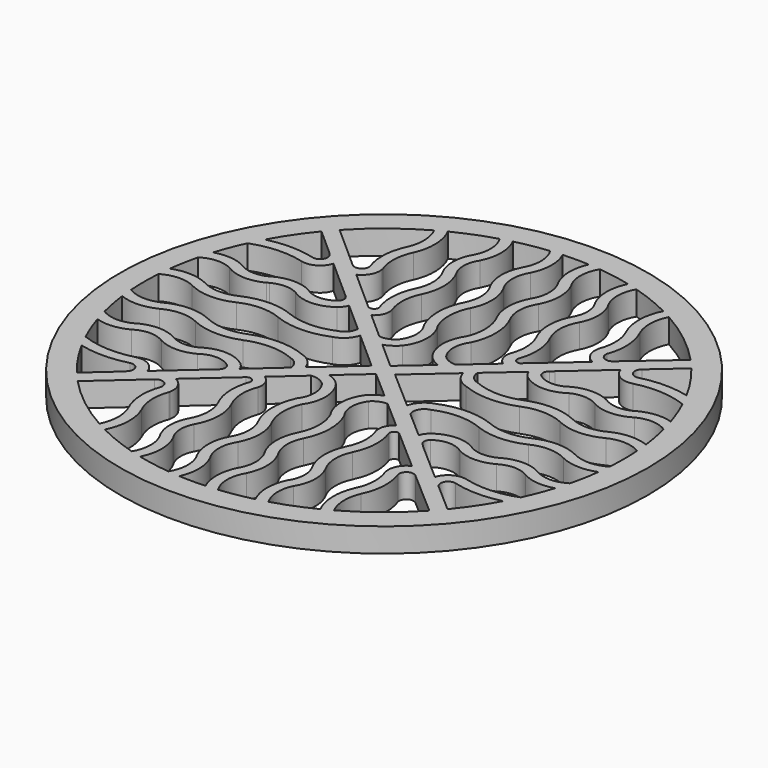
from build123d import *

# Parameters (mm, degrees)
F0_R     = 27.94
F1_DEPTH = 2.54


# Not quite as in the source:
# - ends of sketch curves that miss each other by under 0.0002 mm in the source are joined


with BuildPart() as f1:
    # F0 (on Top) → F1 (new body)
    with BuildSketch(Plane.XY):
        Circle(F0_R)
        with BuildLine():
            Line((-18.5704831808, -17.3290840621), (-13.8005321379, -13.098635549))
            ThreePointArc((-13.8005321379, -13.098635549), (-12.906008286, -13.0112132814), (-12.5460925989, -13.8347885801))
            ThreePointArc((-12.5460925989, -13.8347885801), (-12.8977992847, -16.1722814952), (-12.3113500616, -18.4621828096))
            ThreePointArc((-12.3113500616, -18.4621828096), (-11.9533208933, -20.3219772897), (-12.4161624395, -22.1584952169))
            ThreePointArc((-12.4161624395, -22.1584952169), (-15.6803652612, -19.9821456624), (-18.5704831808, -17.3290840621))
        make_face(mode=Mode.SUBTRACT)
        with BuildLine():
            Line((-16.5311535001, -13.4369904456), (-16.6220914229, -13.564037606))
            Line((-16.6220914229, -13.564037606), (-19.5763440963, -16.1841512543))
            ThreePointArc((-19.5763440963, -16.1841512543), (-21.0445692163, -14.2227320336), (-22.3169864748, -12.1289783034))
            ThreePointArc((-22.3169864748, -12.1289783034), (-19.7773206943, -12.4353403441), (-17.2424184103, -12.0917848367))
            ThreePointArc((-17.2424184103, -12.0917848367), (-16.3555594533, -12.4835065865), (-16.5311535001, -13.4369904456))
        make_face(mode=Mode.SUBTRACT)
        with BuildLine():
            Line((-12.4929334647, -11.9389320609), (-8.1518250801, -8.0888222075))
            ThreePointArc((-8.1518250801, -8.0888222075), (-7.5848144389, -8.0278903633), (-7.3414510498, -8.5436306251))
            ThreePointArc((-7.3414510498, -8.5436306251), (-7.6962049281, -10.8285786216), (-7.1160036617, -13.0669271539))
            ThreePointArc((-7.1160036617, -13.0669271539), (-6.7161500742, -14.9429747655), (-7.2321257599, -16.7904613349))
            ThreePointArc((-7.2321257599, -16.7904613349), (-7.7064237742, -18.845016734), (-7.0859523066, -20.8602516215))
            ThreePointArc((-7.0859523066, -20.8602516215), (-6.7211428867, -22.6227957974), (-7.2321257599, -24.3486417895))
            ThreePointArc((-7.2321257599, -24.3486417895), (-9.3559303924, -23.6141179486), (-11.4065002981, -22.6947516168))
            ThreePointArc((-11.4065002981, -22.6947516168), (-10.8107716851, -20.3540767822), (-11.2731624395, -17.9834553338))
            ThreePointArc((-11.2731624395, -17.9834553338), (-11.758060909, -16.0759793316), (-11.437578849, -14.1341033124))
            Line((-11.437578849, -14.1341033124), (-11.4188391308, -14.0269326452))
            ThreePointArc((-11.4188391308, -14.0269326452), (-11.596606163, -12.7981140346), (-12.4929334647, -11.9389320609))
        make_face(mode=Mode.SUBTRACT)
        with BuildLine():
            Line((-6.9854120479, -7.0543356408), (-4.1093686564, -4.5035854592))
            ThreePointArc((-4.1093686564, -4.5035854592), (-3.2193987681, -4.622483985), (-2.4732761203, -5.1219679745))
            ThreePointArc((-2.4732761203, -5.1219679745), (-1.9512402498, -6.7679594308), (-2.4983765115, -8.4057784791))
            ThreePointArc((-2.4983765115, -8.4057784791), (-3.0543737307, -11.0452272125), (-2.4107500728, -13.6646872925))
            ThreePointArc((-2.4107500728, -13.6646872925), (-2.0125173354, -15.4777115994), (-2.5659752822, -17.2495272647))
            ThreePointArc((-2.5659752822, -17.2495272647), (-3.0984296295, -19.3613287647), (-2.6085446443, -21.4834093261))
            ThreePointArc((-2.6085446443, -21.4834093261), (-2.088534568, -23.3762023641), (-2.6272335105, -25.2637614793))
            ThreePointArc((-2.6272335105, -25.2637614793), (-4.3733190571, -25.020673061), (-6.0983371667, -24.657053429))
            ThreePointArc((-6.0983371667, -24.657053429), (-6.0937218208, -24.6479307461), (-6.0891257599, -24.638798332))
            ThreePointArc((-6.0891257599, -24.638798332), (-5.5749024675, -22.4680644679), (-6.0891257599, -20.2973306037))
            ThreePointArc((-6.0891257599, -20.2973306037), (-6.5627915104, -18.8369130713), (-6.2289017722, -17.3383483398))
            ThreePointArc((-6.2289017722, -17.3383483398), (-5.5734089799, -14.9687958695), (-6.0891257599, -12.5649477228))
            ThreePointArc((-6.0891257599, -12.5649477228), (-6.5561181002, -10.7393618485), (-6.2466127495, -8.8805848129))
            ThreePointArc((-6.2466127495, -8.8805848129), (-6.3100290028, -7.8436762867), (-6.9854120479, -7.0543356408))
        make_face(mode=Mode.SUBTRACT)
        with BuildLine():
            Line((-10.7794748619, -8.3822467826), (-15.2007910101, -12.3034925472))
            ThreePointArc((-15.2007910101, -12.3034925472), (-16.1010101713, -11.1724173912), (-17.5346267563, -10.9867590113))
            ThreePointArc((-17.5346267563, -10.9867590113), (-20.3062535778, -11.2809984553), (-23.0334956908, -10.7059831993))
            ThreePointArc((-23.0334956908, -10.7059831993), (-23.6783363344, -9.19219171), (-24.2238119338, -7.639825613))
            ThreePointArc((-24.2238119338, -7.639825613), (-22.5093516319, -7.8291197338), (-20.856343234, -7.3364031546))
            ThreePointArc((-20.856343234, -7.3364031546), (-19.2961519486, -6.8658747452), (-17.7295057945, -7.3144432007))
            ThreePointArc((-17.7295057945, -7.3144432007), (-15.8135280217, -7.7981545882), (-13.8921396836, -7.3364031546))
            ThreePointArc((-13.8921396836, -7.3364031546), (-12.3358072727, -6.8157514758), (-10.7794748619, -7.3364031546))
            ThreePointArc((-10.7794748619, -7.3364031546), (-10.5312463908, -7.8303040534), (-10.7360509039, -8.3437342659))
            ThreePointArc((-10.7360509039, -8.3437342659), (-10.7573480268, -8.3634582863), (-10.7794748619, -8.3822467826))
        make_face(mode=Mode.SUBTRACT)
        with BuildLine():
            ThreePointArc((-24.6333464508, -6.1934031546), (-24.9649839092, -4.6807668616), (-25.2038268228, -3.1507322145))
            ThreePointArc((-25.2038268228, -3.1507322145), (-23.2746663282, -3.4703434645), (-21.3780211987, -2.994372018))
            ThreePointArc((-21.3780211987, -2.994372018), (-19.501415105, -2.5043500763), (-17.6065823104, -2.9183314944))
            ThreePointArc((-17.6065823104, -2.9183314944), (-15.0565101754, -3.5137315462), (-12.4770380559, -3.0624082698))
            ThreePointArc((-12.4770380559, -3.0624082698), (-9.9451402811, -2.5677176934), (-7.4211004148, -3.1010542307))
            ThreePointArc((-7.4211004148, -3.1010542307), (-6.6509483041, -3.5810685005), (-6.317788309, -4.4251966842))
            Line((-6.317788309, -4.4251966842), (-9.495253242, -7.2432762998))
            ThreePointArc((-9.495253242, -7.2432762998), (-9.7298232295, -6.7980281825), (-10.0775378412, -6.4342102148))
            Line((-10.0775378412, -6.4342102148), (-10.0916950959, -6.4234913333))
            ThreePointArc((-10.0916950959, -6.4234913333), (-12.2793958042, -5.673178142), (-14.4887914077, -6.3569729516))
            ThreePointArc((-14.4887914077, -6.3569729516), (-15.9583042621, -6.6504710139), (-17.3854335884, -6.1934031546))
            ThreePointArc((-17.3854335884, -6.1934031546), (-19.4293945717, -5.7257275396), (-21.4318401679, -6.3475865402))
            ThreePointArc((-21.4318401679, -6.3475865402), (-23.0532754063, -6.6999436052), (-24.6333464508, -6.1934031546))
        make_face(mode=Mode.SUBTRACT)
        with BuildLine():
            Line((-3.0008579849, -3.4897487406), (-0.1074668487, -0.9299076392))
            Line((-0.1074668487, -0.9299076392), (2.8724846558, -3.5323386056))
            ThreePointArc((2.8724846558, -3.5323386056), (2.1752585082, -3.8839965102), (1.5870080755, -4.397561512))
            ThreePointArc((1.5870080755, -4.397561512), (0.8087695638, -6.6735323176), (1.5017849321, -8.9768837863))
            ThreePointArc((1.5017849321, -8.9768837863), (1.9103804325, -11.0743224779), (1.3914487995, -13.1472212473))
            ThreePointArc((1.3914487995, -13.1472212473), (1.3803900845, -13.1691739034), (1.3692218584, -13.1910710497))
            ThreePointArc((1.3692218584, -13.1910710497), (0.8667364927, -15.4065827451), (1.4482800878, -17.602668049))
            Line((1.4482800878, -17.602668049), (1.4530981237, -17.6022709756))
            ThreePointArc((1.4530981237, -17.6022709756), (1.955462941, -19.4080288753), (1.4530232551, -21.2137659447))
            ThreePointArc((1.4530232551, -21.2137659447), (0.9458843119, -23.2802576622), (1.385342962, -25.3621928247))
            ThreePointArc((1.385342962, -25.3621928247), (-0.0001316396, -25.3999999997), (-1.3856058492, -25.3621784638))
            ThreePointArc((-1.3856058492, -25.3621784638), (-0.9461256192, -23.2802478565), (-1.4532431425, -21.2137508825))
            ThreePointArc((-1.4532431425, -21.2137508825), (-1.9554739954, -19.3715116674), (-1.4149317469, -17.5401473582))
            ThreePointArc((-1.4149317469, -17.5401473582), (-0.8661983565, -15.3465313443), (-1.3915850746, -13.1472068237))
            ThreePointArc((-1.3915850746, -13.1472068237), (-1.9104952213, -11.0743026756), (-1.5018779803, -8.9768682194))
            ThreePointArc((-1.5018779803, -8.9768682194), (-0.8088387371, -6.6735239341), (-1.5870536575, -4.3975450619))
            ThreePointArc((-1.5870536575, -4.3975450619), (-2.2317910283, -3.8468312927), (-3.0008579849, -3.4897487406))
        make_face(mode=Mode.SUBTRACT)
        with BuildLine():
            ThreePointArc((-7.0508121213, 2.0164165737), (-6.0285782094, 2.6143373536), (-5.4245050427, 3.6329477006))
            Line((-5.4245050427, 3.6329477006), (-1.328253163, 0))
            Line((-1.328253163, 0), (-5.4245050427, -3.6329477006))
            ThreePointArc((-5.4245050427, -3.6329477006), (-6.0285782094, -2.6143373536), (-7.0508121213, -2.0164165737))
            ThreePointArc((-7.0508121213, -2.0164165737), (-9.9151064709, -1.4249436512), (-12.7911253305, -1.9564865542))
            ThreePointArc((-12.7911253305, -1.9564865542), (-14.9632901191, -2.3725531643), (-17.1202818141, -1.8838834183))
            ThreePointArc((-17.1202818141, -1.8838834183), (-19.5178722599, -1.3614536781), (-21.8939850089, -1.9742023898))
            ThreePointArc((-21.8939850089, -1.9742023898), (-23.6334472472, -2.3277315026), (-25.3346326389, -1.8210955631))
            ThreePointArc((-25.3346326389, -1.8210955631), (-25.4, 0), (-25.3346326389, 1.8210955631))
            ThreePointArc((-25.3346326389, 1.8210955631), (-23.6334472472, 2.3277315026), (-21.8939850089, 1.9742023898))
            ThreePointArc((-21.8939850089, 1.9742023898), (-19.5178722599, 1.3614536781), (-17.1202818141, 1.8838834183))
            ThreePointArc((-17.1202818141, 1.8838834183), (-14.9632901191, 2.3725531643), (-12.7911253305, 1.9564865542))
            ThreePointArc((-12.7911253305, 1.9564865542), (-9.9151064709, 1.4249436512), (-7.0508121213, 2.0164165737))
        make_face(mode=Mode.SUBTRACT)
        with BuildLine():
            ThreePointArc((2.4732230294, -5.1219936106), (3.1568867484, -4.6473445579), (3.9751637063, -4.4953227692))
            Line((3.9751637063, -4.4953227692), (6.9387020687, -7.083419922))
            ThreePointArc((6.9387020687, -7.083419922), (6.2571533754, -7.995229289), (6.3360513806, -9.1308700983))
            ThreePointArc((6.3360513806, -9.1308700983), (6.548399798, -10.8721037819), (6.0889955199, -12.5650108379))
            ThreePointArc((6.0889955199, -12.5650108379), (5.5732538232, -14.9688536389), (6.2287220543, -17.3384129034))
            ThreePointArc((6.2287220543, -17.3384129034), (6.5625962594, -18.8369810958), (6.0889153712, -20.2973937184))
            ThreePointArc((6.0889153712, -20.2973937184), (5.5746802731, -22.4783459819), (6.0980815881, -24.6571166389))
            ThreePointArc((6.0980815881, -24.6571166389), (4.3733190571, -25.020673061), (2.6274953773, -25.2637342458))
            ThreePointArc((2.6274953773, -25.2637342458), (2.6272335106, -25.2637614793), (2.6269716436, -25.26378871))
            ThreePointArc((2.6269716436, -25.26378871), (2.0882922662, -23.3762240111), (2.6083219619, -21.4834363632))
            ThreePointArc((2.6083219619, -21.4834363632), (3.0982289432, -19.3613608798), (2.5657964854, -17.2495538608))
            ThreePointArc((2.5657964852, -17.2495538609), (2.0123569038, -15.477732459), (2.4106084338, -13.66471228))
            ThreePointArc((2.4106084338, -13.66471228), (3.0542592432, -11.0452588714), (2.4982893827, -8.4058043752))
            ThreePointArc((2.4982893827, -8.4058043752), (1.9511700977, -6.7679796556), (2.4732230294, -5.1219936106))
        make_face(mode=Mode.SUBTRACT)
        with BuildLine():
            ThreePointArc((7.3413624919, -8.5437067211), (7.5012043652, -8.0870491747), (7.9748425974, -7.9882951165))
            Line((7.9748425974, -7.9882951165), (12.4966825061, -11.9372775699))
            ThreePointArc((12.4966825061, -11.9372775699), (11.597449826, -12.7963389578), (11.4186937366, -14.0270510044))
            Line((11.4186937366, -14.0270510044), (11.4374323439, -14.1342218658))
            ThreePointArc((11.4374323439, -14.1342218658), (11.7578942757, -16.0761012068), (11.2729760346, -17.9835721827))
            ThreePointArc((11.2729760346, -17.9835721827), (10.810560708, -20.3541888383), (11.4062650591, -22.6948698477))
            ThreePointArc((11.4062650591, -22.6948698477), (9.355685624, -23.6142149246), (7.231873378, -24.3487167515))
            ThreePointArc((7.231873378, -24.3487167515), (6.7209083938, -22.622865463), (7.0857360831, -20.8603250686))
            ThreePointArc((7.0857360831, -20.8603250686), (7.7062284391, -18.8450966125), (7.231951721, -16.7905362973))
            ThreePointArc((7.231951721, -16.7905362973), (6.7159951852, -14.9430443797), (7.1158682184, -13.0670009128))
            ThreePointArc((7.1158682184, -13.0670009128), (7.696092686, -10.8286583947), (7.3413624919, -8.5437067211))
        make_face(mode=Mode.SUBTRACT)
        with BuildLine():
            ThreePointArc((18.6153947957, -17.2808297428), (15.7061784481, -19.9618626024), (12.4159327589, -22.1586239132))
            ThreePointArc((12.4159327589, -22.1586239132), (11.9531102489, -20.3221011886), (12.3111586945, -18.4623104196))
            ThreePointArc((12.3111586945, -18.4623104196), (12.8976316531, -16.1724151841), (12.5459491962, -13.8349186236))
            ThreePointArc((12.5459491962, -13.8349186236), (12.90587342, -13.0113470556), (13.8003963656, -13.0987785953))
            Line((13.8003963656, -13.0987785953), (18.6153947957, -17.2808297428))
        make_face(mode=Mode.SUBTRACT)
        with BuildLine():
            ThreePointArc((22.3168607528, -12.1292096255), (21.0629293857, -14.1955276651), (19.6182702445, -16.1333032146))
            Line((19.6182702445, -16.1333032146), (16.5310142205, -13.4371617956))
            ThreePointArc((16.5310142205, -13.4371617956), (16.3554300569, -12.4836761164), (17.2422930741, -12.0919635592))
            ThreePointArc((17.2422930741, -12.0919635592), (19.777191797, -12.4355453417), (22.3168607528, -12.1292096255))
        make_face(mode=Mode.SUBTRACT)
        with BuildLine():
            Line((1.1805804842, -0.0314254801), (5.4112533657, 3.6805990737))
            ThreePointArc((5.4112533657, 3.6805990737), (6.0111348367, 2.6318235073), (7.0508330218, 2.0163434897))
            ThreePointArc((7.0508330218, 2.0163434897), (9.9151212403, 1.4248408779), (12.7911456094, 1.95635397))
            ThreePointArc((12.7911456094, 1.95635397), (14.9633147106, 2.3723980649), (17.1203013402, 1.883705961))
            ThreePointArc((17.1203013402, 1.883705961), (19.5178863708, 1.3612513691), (21.894005471, 1.9739754515))
            ThreePointArc((21.894005471, 1.9739754515), (23.6334713736, 2.3274865343), (25.3346515138, 1.8208329614))
            ThreePointArc((25.3346515138, 1.8208329614), (25.4, 0), (25.3346515138, -1.8208329614))
            ThreePointArc((25.3346515138, -1.8208329614), (23.6334713736, -2.3274865343), (21.894005471, -1.9739754515))
            ThreePointArc((21.894005471, -1.9739754515), (19.5178863708, -1.3612513691), (17.1203013402, -1.883705961))
            ThreePointArc((17.1203013402, -1.883705961), (14.9633147106, -2.3723980649), (12.7911456094, -1.95635397))
            ThreePointArc((12.7911456094, -1.95635397), (9.9151212403, -1.4248408779), (7.0508330218, -2.0163434897))
            ThreePointArc((7.0508330218, -2.0163434897), (5.9977288514, -2.6455421173), (5.4016477625, -3.717739227))
            Line((5.4016477625, -3.717739227), (1.1805804842, -0.0314254801))
        make_face(mode=Mode.SUBTRACT)
        with BuildLine():
            ThreePointArc((17.5345128741, -10.9869407627), (16.1110985529, -11.1668680867), (15.2074294336, -12.2812577378))
            Line((15.2074294336, -12.2812577378), (11.1406161812, -8.7296560669))
            Line((11.1406161812, -8.7296560669), (10.7793879767, -8.3823585148))
            ThreePointArc((10.7793879767, -8.3823585148), (10.5305397004, -7.8594341214), (10.7793988172, -7.3365148869))
            ThreePointArc((10.7793988172, -7.3365148869), (12.3357366246, -6.81587934), (13.8920636387, -7.3365471507))
            ThreePointArc((13.8920636387, -7.3365471507), (15.8134471905, -7.7983185001), (17.729429977, -7.3146269723))
            ThreePointArc((17.729429977, -7.3146269723), (19.2960807805, -6.8660747556), (20.8562671887, -7.3366193369))
            ThreePointArc((20.8562671887, -7.3366193369), (22.5092704794, -7.82935305), (24.2237327433, -7.6400767001))
            ThreePointArc((24.2237327433, -7.6400767001), (23.6782410532, -9.192437143), (23.0333847186, -10.7062219482))
            ThreePointArc((23.0333847186, -10.7062219482), (20.3061366455, -11.2812089355), (17.5345128741, -10.9869407627))
        make_face(mode=Mode.SUBTRACT)
        with BuildLine():
            Line((9.4820197072, -7.2811818828), (6.5530349027, -4.7232608079))
            ThreePointArc((6.5530349027, -4.7232608079), (6.6185456375, -3.7149112001), (7.4211325578, -3.1009773085))
            ThreePointArc((7.4211325578, -3.1009773085), (9.9451668958, -2.5676146087), (12.477069798, -3.0622789412))
            ThreePointArc((12.477069798, -3.0622789412), (15.0565465956, -3.5135754804), (17.6066125589, -2.9181489964))
            ThreePointArc((17.6066125589, -2.9181489964), (19.5014410624, -2.5041479377), (21.3780522351, -2.9941504278))
            ThreePointArc((21.3780522351, -2.9941504278), (23.2747022981, -3.470102215), (25.2038594798, -3.1504709686))
            ThreePointArc((25.2038594798, -3.1504709686), (24.9649839092, -4.6807668616), (24.6332822529, -6.1936584868))
            ThreePointArc((24.6332822529, -6.1936584868), (23.053205958, -6.7001825594), (21.431774372, -6.3478086878))
            ThreePointArc((21.431774372, -6.3478086878), (19.4293352217, -5.7259289311), (17.3853693908, -6.1935833599))
            ThreePointArc((17.3853693908, -6.1935833599), (15.958235327, -6.6506364265), (14.4887255148, -6.3571231323))
            ThreePointArc((14.4887255148, -6.3571231323), (12.2793369993, -5.6733054215), (10.0916285138, -6.4235959366))
            Line((10.0916285138, -6.4235959366), (10.077471148, -6.4343146713))
            ThreePointArc((10.077471148, -6.4343146713), (9.7181499836, -6.8144391308), (9.4820197072, -7.2811818828))
        make_face(mode=Mode.SUBTRACT)
        with BuildLine():
            ThreePointArc((-10.1148341299, 6.4056053035), (-9.7436825828, 6.7790435487), (-9.4951932373, 7.2432230819))
            Line((-9.4951932373, 7.2432230819), (-6.317788309, 4.4251966842))
            ThreePointArc((-6.317788309, 4.4251966842), (-6.6509483041, 3.5810685005), (-7.4211004148, 3.1010542307))
            ThreePointArc((-7.4211004148, 3.1010542307), (-9.8831598487, 2.5684882175), (-12.3620960269, 3.0159685396))
            ThreePointArc((-12.3620960269, 3.0159685396), (-14.9945418636, 3.5151786201), (-17.6065823104, 2.9183314944))
            ThreePointArc((-17.6065823104, 2.9183314944), (-19.501415105, 2.5043500763), (-21.3780211987, 2.994372018))
            ThreePointArc((-21.3780211987, 2.994372018), (-23.2746663282, 3.4703434645), (-25.2038268228, 3.1507322145))
            ThreePointArc((-25.2038268228, 3.1507322145), (-24.9649353902, 4.6810256314), (-24.6332180523, 6.1939138183))
            ThreePointArc((-24.6332180523, 6.1939138183), (-23.0531365072, 6.7004215129), (-21.4317085738, 6.3480308346))
            ThreePointArc((-21.4317085738, 6.3480308346), (-19.4254245013, 5.7259853337), (-17.3784999898, 6.1973837102))
            ThreePointArc((-17.3784999898, 6.1973837102), (-17.2739491044, 6.2601253131), (-17.1669247978, 6.3185478616))
            ThreePointArc((-17.1669247978, 6.3185478616), (-15.8321543672, 6.6547898981), (-14.4883225858, 6.3568185018))
            ThreePointArc((-14.4883225858, 6.3568185018), (-12.2936757621, 5.6727844094), (-10.1148341299, 6.4056053035))
        make_face(mode=Mode.SUBTRACT)
        with BuildLine():
            ThreePointArc((-17.53439899, 10.987122513), (-16.1009733187, 11.1726413097), (-15.2006627532, 12.3033787968))
            Line((-15.2006627532, 12.3033787968), (-11.2678816749, 8.8154126279))
            Line((-11.2678816749, 8.8154126279), (-10.7793010903, 8.3824702462))
            ThreePointArc((-10.7793010903, 8.3824702462), (-10.5304582343, 7.8595432734), (-10.7793227713, 7.3366266184))
            ThreePointArc((-10.7793227713, 7.3366266184), (-12.3356659752, 6.8160072035), (-13.8919875922, 7.336691146))
            ThreePointArc((-13.8919875922, 7.336691146), (-15.8133663576, 7.7984824111), (-17.7293541576, 7.3148107432))
            ThreePointArc((-17.7293541576, 7.3148107432), (-19.2960096104, 6.8662747653), (-20.8561911412, 7.3368355184))
            ThreePointArc((-20.8561911412, 7.3368355184), (-22.5091893244, 7.8295863653), (-24.2236535501, 7.6403277864))
            ThreePointArc((-24.2236535501, 7.6403277864), (-23.6781457693, 9.1926825751), (-23.0332737439, 10.7064606961))
            ThreePointArc((-23.0332737439, 10.7064606961), (-20.3060197111, 11.2814194145), (-17.53439899, 10.987122513))
        make_face(mode=Mode.SUBTRACT)
        with BuildLine():
            Line((-0.0935980345, 0.9420194576), (-2.9752503048, 3.497744129))
            ThreePointArc((-2.9752503048, 3.497744129), (-2.2205142055, 3.8540970497), (-1.5870455095, 4.3975410624))
            ThreePointArc((-1.5870455095, 4.3975410624), (-0.8088387371, 6.6735239341), (-1.5018779803, 8.9768682194))
            ThreePointArc((-1.5018779803, 8.9768682194), (-1.9104952213, 11.0743026756), (-1.3915850746, 13.1472068237))
            ThreePointArc((-1.3915850746, 13.1472068237), (-0.8661983565, 15.3465313443), (-1.4149317469, 17.5401473582))
            ThreePointArc((-1.4149317469, 17.5401473582), (-1.9554739954, 19.3715116674), (-1.4532431425, 21.2137508825))
            ThreePointArc((-1.4532431425, 21.2137508825), (-0.9461256192, 23.2802478565), (-1.3856058492, 25.3621784638))
            ThreePointArc((-1.3856058492, 25.3621784638), (0.0001316396, 25.3999999997), (1.3858687362, 25.3621641002))
            ThreePointArc((1.3858687362, 25.3621641002), (0.9463669263, 23.2802380484), (1.4534630297, 21.213735818))
            ThreePointArc((1.4534630297, 21.213735818), (1.9557189614, 19.4399749856), (1.4860006972, 17.6573215522))
            Line((1.4860006972, 17.6573215522), (1.448645002, 17.6026380215))
            ThreePointArc((1.448645002, 17.6026380215), (0.8670558808, 15.4065647738), (1.3694953175, 13.191042662))
            ThreePointArc((1.3694953175, 13.191042662), (1.9098990397, 11.0988533587), (1.5019710284, 8.9768526514))
            ThreePointArc((1.5019710284, 8.9768526514), (0.8089079102, 6.6735155499), (1.5870992394, 4.3975286113))
            ThreePointArc((1.5870992394, 4.3975286113), (2.1752947902, 3.8839811904), (2.8724574089, 3.5323148105))
            Line((2.8724574089, 3.5323148105), (-0.0935980345, 0.9420194576))
        make_face(mode=Mode.SUBTRACT)
        with BuildLine():
            ThreePointArc((-22.3167350285, 12.1294409462), (-21.044421792, 14.2229501665), (-19.5763440963, 16.1841512543))
            Line((-19.5763440963, 16.1841512543), (-16.6362890902, 13.5766294544))
            Line((-16.6362890902, 13.5766294544), (-16.5308749391, 13.4373331441))
            ThreePointArc((-16.5308749391, 13.4373331441), (-16.3553006587, 12.483845645), (-17.2421677361, 12.0921422805))
            ThreePointArc((-17.2421677361, 12.0921422805), (-19.7770628975, 12.4357503379), (-22.3167350285, 12.1294409462))
        make_face(mode=Mode.SUBTRACT)
        with BuildLine():
            ThreePointArc((-18.5704831808, 17.3290840621), (-15.680158139, 19.9823081934), (-12.415703077, 22.1587526071))
            ThreePointArc((-12.415703077, 22.1587526071), (-11.9528996031, 20.3222250853), (-12.3109673261, 18.4624380278))
            ThreePointArc((-12.3109673261, 18.4624380278), (-12.8974640201, 16.1725488713), (-12.5458057922, 13.8350486656))
            ThreePointArc((-12.5458057922, 13.8350486656), (-12.9057385525, 13.0114808284), (-13.8002605919, 13.0989216401))
            Line((-13.8002605919, 13.0989216401), (-18.5704831808, 17.3290840621))
        make_face(mode=Mode.SUBTRACT)
        with BuildLine():
            Line((-8.151816932, 8.0888182079), (-12.4930325787, 11.9390231915))
            ThreePointArc((-12.4930325787, 11.9390231915), (-11.5964220901, 12.7981766958), (-11.4185401931, 14.0271653625))
            Line((-11.4185401931, 14.0271653625), (-11.4372858375, 14.1343404177))
            ThreePointArc((-11.4372858375, 14.1343404177), (-11.7577276411, 16.0762230803), (-11.2727896285, 17.9836890298))
            ThreePointArc((-11.2727896285, 17.9836890298), (-10.8103497297, 20.3543008921), (-11.4060298189, 22.694988076))
            ThreePointArc((-11.4060298189, 22.694988076), (-9.3557040755, 23.6142076143), (-7.2321638106, 24.3486304875))
            ThreePointArc((-7.2321638106, 24.3486304875), (-6.7209091166, 22.6227254826), (-7.0855726054, 20.8600145058))
            ThreePointArc((-7.0855726054, 20.8600145058), (-7.6994050021, 18.8463966474), (-7.2220009663, 16.796144839))
            ThreePointArc((-7.2220009663, 16.796144839), (-6.7095493857, 14.9413227032), (-7.1188817231, 13.0610517611))
            ThreePointArc((-7.1188817231, 13.0610517611), (-7.6963586844, 10.8253074133), (-7.3414429017, 8.5436266255))
            ThreePointArc((-7.3414429017, 8.5436266255), (-7.5848062909, 8.0278863637), (-8.151816932, 8.0888182079))
        make_face(mode=Mode.SUBTRACT)
        with BuildLine():
            Line((-4.1093605084, 4.5035814597), (-6.9854038998, 7.0543316412))
            ThreePointArc((-6.9854038998, 7.0543316412), (-6.3100208547, 7.8436722871), (-6.2466046015, 8.8805808133))
            ThreePointArc((-6.2466046015, 8.8805808133), (-6.5562874842, 10.7351592817), (-6.0928279532, 12.5574024176))
            ThreePointArc((-6.0928279532, 12.5574024176), (-5.5668049267, 14.9661974334), (-6.2187820407, 17.3439946273))
            ThreePointArc((-6.2187820407, 17.3439946273), (-6.5558288499, 18.8393593766), (-6.0877699501, 20.2990295967))
            ThreePointArc((-6.0877699501, 20.2990295967), (-5.5746648264, 22.4792984795), (-6.0983395303, 24.6570528444))
            ThreePointArc((-6.0983395303, 24.6570528444), (-4.3733202563, 25.0206728514), (-2.6272335105, 25.2637614793))
            ThreePointArc((-2.6272335105, 25.2637614793), (-2.088534568, 23.3762023641), (-2.6085446443, 21.4834093261))
            ThreePointArc((-2.6085446443, 21.4834093261), (-3.0984296295, 19.3613287647), (-2.5659752822, 17.2495272647))
            ThreePointArc((-2.5659752822, 17.2495272647), (-2.0125173354, 15.4777115994), (-2.4107500728, 13.6646872925))
            ThreePointArc((-2.4107500728, 13.6646872925), (-3.0543737307, 11.0452272125), (-2.4983765115, 8.4057784791))
            ThreePointArc((-2.4983765115, 8.4057784791), (-1.9512402498, 6.7679594308), (-2.4732761203, 5.1219679745))
            ThreePointArc((-2.4732761203, 5.1219679745), (-3.2193906201, 4.6224799854), (-4.1093605084, 4.5035814597))
        make_face(mode=Mode.SUBTRACT)
        with BuildLine():
            ThreePointArc((12.477069798, 3.0622789412), (9.9451668958, 2.5676146087), (7.4211325578, 3.1009773085))
            ThreePointArc((7.4211325578, 3.1009773085), (6.6353939452, 3.6000388062), (6.315859227, 4.4743071344))
            Line((6.315859227, 4.4743071344), (9.4896280116, 7.2589959975))
            ThreePointArc((9.4896280116, 7.2589959975), (9.7249260856, 6.8048677765), (10.077471148, 6.4343146713))
            Line((10.077471148, 6.4343146713), (10.0916285138, 6.4235959366))
            ThreePointArc((10.0916285138, 6.4235959366), (12.2793369993, 5.6733054215), (14.4887255148, 6.3571231323))
            ThreePointArc((14.4887255148, 6.3571231323), (15.958235327, 6.6506364265), (17.3853693908, 6.1935833599))
            ThreePointArc((17.3853693908, 6.1935833599), (19.4293352217, 5.7259289311), (21.431774372, 6.3478086878))
            ThreePointArc((21.431774372, 6.3478086878), (23.053205958, 6.7001825594), (24.6332822529, 6.1936584868))
            ThreePointArc((24.6332822529, 6.1936584868), (24.9649839092, 4.6807668616), (25.2038594798, 3.1504709686))
            ThreePointArc((25.2038594798, 3.1504709686), (23.2747022981, 3.470102215), (21.3780522351, 2.9941504278))
            ThreePointArc((21.3780522351, 2.9941504278), (19.5014410624, 2.5041479377), (17.6066125589, 2.9181489964))
            ThreePointArc((17.6066125589, 2.9181489964), (15.0565465956, 3.5135754804), (12.477069798, 3.0622789412))
        make_face(mode=Mode.SUBTRACT)
        with BuildLine():
            Line((11.1451711317, 8.7115821188), (15.2087504005, 12.2769974662))
            ThreePointArc((15.2087504005, 12.2769974662), (16.1147224519, 11.164857589), (17.5382151623, 10.987914186))
            ThreePointArc((17.5382151623, 10.987914186), (20.3166874731, 11.2695155619), (23.0461746743, 10.6786625042))
            ThreePointArc((23.0461746743, 10.6786625042), (23.6837346662, 9.178273926), (24.2237327433, 7.6400767001))
            ThreePointArc((24.2237327433, 7.6400767001), (22.5092704794, 7.82935305), (20.8562671887, 7.3366193369))
            ThreePointArc((20.8562671887, 7.3366193369), (19.2960807805, 6.8660747556), (17.729429977, 7.3146269723))
            ThreePointArc((17.729429977, 7.3146269723), (15.8134471905, 7.7983185001), (13.8920636387, 7.3365471507))
            ThreePointArc((13.8920636387, 7.3365471507), (12.3357366246, 6.81587934), (10.7793988172, 7.3365148869))
            ThreePointArc((10.7793988172, 7.3365148869), (10.5305397004, 7.8594341214), (10.7793879767, 8.3823585148))
            Line((10.7793879767, 8.3823585148), (11.1451711317, 8.7115821188))
        make_face(mode=Mode.SUBTRACT)
        with BuildLine():
            ThreePointArc((6.2465206991, 8.8806495605), (6.2998624206, 7.8692860006), (6.9387020687, 7.083419922))
            Line((6.9387020687, 7.083419922), (3.9750631671, 4.495234967))
            ThreePointArc((3.9750631671, 4.495234967), (3.156893662, 4.6473164304), (2.473329211, 5.121942338))
            ThreePointArc((2.473329211, 5.121942338), (1.9513104018, 6.7679392052), (2.4984636399, 8.4057525822))
            ThreePointArc((2.4984636399, 8.4057525822), (3.0544882178, 11.0451955523), (2.4108917115, 13.6646623036))
            ThreePointArc((2.4108917115, 13.6646623036), (2.0126777667, 15.4776907382), (2.566154079, 17.2495006666))
            ThreePointArc((2.566154079, 17.2495006666), (3.0986303157, 19.3612966475), (2.6087673266, 21.4833822865))
            Line((2.6087673266, 21.4833822865), (2.598689527, 21.500253207))
            ThreePointArc((2.598689527, 21.500253207), (2.088838811, 23.386006387), (2.6274953773, 25.2637342458))
            ThreePointArc((2.6274953773, 25.2637342458), (4.3733190571, 25.020673061), (6.0980815881, 24.6571166389))
            ThreePointArc((6.0980815881, 24.6571166389), (5.5746802731, 22.4783459819), (6.0889153712, 20.2973937184))
            ThreePointArc((6.0889153712, 20.2973937184), (6.5625962594, 18.8369810958), (6.2287220543, 17.3384129034))
            ThreePointArc((6.2287220543, 17.3384129034), (5.5732538232, 14.9688536389), (6.0889955199, 12.5650108379))
            ThreePointArc((6.0889955199, 12.5650108379), (6.5560067829, 10.7394298042), (6.2465206991, 8.8806495605))
        make_face(mode=Mode.SUBTRACT)
        with BuildLine():
            ThreePointArc((7.231873378, 24.3487167515), (9.355685624, 23.6142149246), (11.4062650591, 22.6948698477))
            ThreePointArc((11.4062650591, 22.6948698477), (10.810560708, 20.3541888383), (11.2729760346, 17.9835721827))
            ThreePointArc((11.2729760346, 17.9835721827), (11.7578942757, 16.0761012068), (11.4374323439, 14.1342218658))
            Line((11.4374323439, 14.1342218658), (11.4186937366, 14.0270510044))
            ThreePointArc((11.4186937366, 14.0270510044), (11.597449826, 12.7963389578), (12.4966825061, 11.9372775699))
            Line((12.4966825061, 11.9372775699), (8.0190896661, 8.0269366654))
            Line((8.0190896661, 8.0269366654), (7.9748425974, 7.9882951165))
            ThreePointArc((7.9748425974, 7.9882951165), (7.5012043652, 8.0870491747), (7.3413624919, 8.5437067211))
            ThreePointArc((7.3413624919, 8.5437067211), (7.696092686, 10.8286583947), (7.1158682184, 13.0670009128))
            ThreePointArc((7.1158682184, 13.0670009128), (6.7159951852, 14.9430443797), (7.231951721, 16.7905362973))
            ThreePointArc((7.231951721, 16.7905362973), (7.7062284391, 18.8450966125), (7.0857360831, 20.8603250686))
            ThreePointArc((7.0857360831, 20.8603250686), (6.7209083938, 22.622865463), (7.231873378, 24.3487167515))
        make_face(mode=Mode.SUBTRACT)
        with BuildLine():
            Line((16.5310142205, 13.4371617956), (19.6122307012, 16.1406445635))
            ThreePointArc((19.6122307012, 16.1406445635), (21.06696281, 14.1895411471), (22.3282844855, 12.1081671584))
            ThreePointArc((22.3282844855, 12.1081671584), (19.7864087569, 12.4265060131), (17.2464714009, 12.0930542575))
            ThreePointArc((17.2464714009, 12.0930542575), (16.3564419592, 12.4817687434), (16.5310142205, 13.4371617956))
        make_face(mode=Mode.SUBTRACT)
        with BuildLine():
            ThreePointArc((12.4159327589, 22.1586239132), (15.7061784481, 19.9618626024), (18.6153947957, 17.2808297428))
            Line((18.6153947957, 17.2808297428), (13.8003963656, 13.0987785953))
            ThreePointArc((13.8003963656, 13.0987785953), (12.90587342, 13.0113470556), (12.5459491962, 13.8349186236))
            ThreePointArc((12.5459491962, 13.8349186236), (12.8976316531, 16.1724151841), (12.3111586945, 18.4623104196))
            ThreePointArc((12.3111586945, 18.4623104196), (11.9531102489, 20.3221011886), (12.4159327589, 22.1586239132))
        make_face(mode=Mode.SUBTRACT)
    extrude(amount=F1_DEPTH)


solid = f1.part
